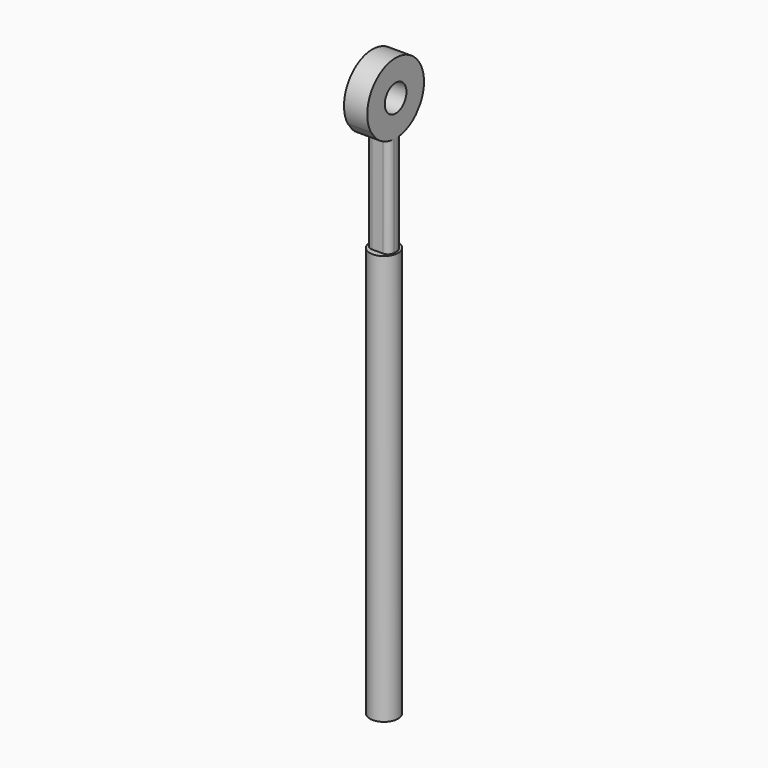
from build123d import *

# Parameters (mm, degrees)
F0_R         = 1.778
F1_DEPTH     = 51.562
F2_W         = 2.9239974657
F2_H         = 2.0237032442
F3_DEPTH     = 12.7
F4_R         = 1.7034886821
F5_DEPTH     = 2.92354
F6_T4_DEPTH  = 14.605
F6_S5_R      = 4.4583340214
F6_T6_DEPTH  = 9
F6_T10_DEPTH = 14.605
F6_S11_R     = 4.4583340214
F6_T12_DEPTH = 9
F6_T16_DEPTH = 14.605
F6_S17_R     = 4.4583340214
F6_T18_DEPTH = 9
F6_T22_DEPTH = 14.605
F6_S23_R     = 4.4583340214
F6_T24_DEPTH = 9


# Not quite as in the source:
# - a fillet or chamfer that OpenCascade refuses, or shapes differently, is made with other operations: its cross-section is extruded or revolved along the edge and cut away or added


with BuildPart() as f1:
    # F0 (on Top) → F1 (new body)
    with BuildSketch(Plane.XY):
        Circle(F0_R)
    extrude(amount=F1_DEPTH)

    # F2 (on face) → F3 (join)
    with BuildSketch(Plane.XY.offset(51.562)):
        Rectangle(F2_W, F2_H)
    extrude(amount=F3_DEPTH)

    # F4 (on face) → F5 (join)
    with BuildSketch(Plane.YZ.offset(1.4619987328)):
        with BuildLine():
            ThreePointArc((3.8834322811, 66.4140847097), (4.3122140778, 67.4719359292), (4.4583340214, 68.6039924622))
            ThreePointArc((4.4583340214, 68.6039924622), (-1.132056533, 72.91620654), (-3.8834322811, 66.4140847097))
            add(Edge.make_bspline(
                [(-3.1221140478, 65.4213605138), (-3.3692442223, 65.7498568477), (-3.6264069605, 66.0819292585), (-3.8834322811, 66.4140847097)],
                knots=[0.8083200784, 0.8083200784, 0.8083200784, 0.8083200784, 1, 1, 1, 1], degree=3))
            ThreePointArc((-3.1221140478, 65.4213605138), (-2.1467294288, 64.6965258908), (-1.0118516221, 64.262))
            Line((-1.0118516221, 64.262), (1.0118516221, 64.262))
            ThreePointArc((1.0118516221, 64.262), (2.1467294288, 64.6965258908), (3.1221140478, 65.4213605138))
            add(Edge.make_bspline(
                [(3.1221140478, 65.4213605138), (3.3692442223, 65.7498568477), (3.6264069605, 66.0819292585), (3.8834322811, 66.4140847097)],
                knots=[0.8083200784, 0.8083200784, 0.8083200784, 0.8083200784, 1, 1, 1, 1], degree=3))
        make_face()
        with Locations((0, 68.6039924622)):
            Circle(F4_R, mode=Mode.SUBTRACT)
    extrude(amount=-F5_DEPTH)

    # F6: fillet of radius 0.762 on 4 edges, made by hand


with BuildPart() as f6_tool2:
    # F6_s3 → F6_t4 (new body)
    with BuildSketch(Plane.XY.offset(51.562)):
        with BuildLine():
            ThreePointArc((1.4619987328, -0.2498516221), (1.2388141001, -0.7886669894), (0.6999987328, -1.0118516221))
            Line((0.6999987328, -1.0118516221), (1.4619987328, -1.0118516221))
            Line((1.4619987328, -1.0118516221), (1.4619987328, -0.2498516221))
        make_face()
    extrude(amount=F6_T4_DEPTH)

    # F6_s5 → F6_t6 (cut, symmetric)
    with BuildSketch(Plane.YZ.offset(1.1)):
        with Locations((0, 68.6039924622)):
            Circle(F6_S5_R)
    extrude(amount=F6_T6_DEPTH, both=True, mode=Mode.SUBTRACT)


with BuildPart() as f1_1:
    add(f1.part)

    # F6_t1: cut F6_tool2
    add(f6_tool2.part, mode=Mode.SUBTRACT)


with BuildPart() as f6_tool8:
    # F6_s9 → F6_t10 (new body)
    with BuildSketch(Plane.XY.offset(51.562)):
        with BuildLine():
            ThreePointArc((-1.4619987328, 0.2498516221), (-1.2388141001, 0.7886669894), (-0.6999987328, 1.0118516221))
            Line((-0.6999987328, 1.0118516221), (-1.4619987328, 1.0118516221))
            Line((-1.4619987328, 1.0118516221), (-1.4619987328, 0.2498516221))
        make_face()
    extrude(amount=F6_T10_DEPTH)

    # F6_s11 → F6_t12 (cut, symmetric)
    with BuildSketch(Plane.YZ.offset(-1.1)):
        with Locations((0, 68.6039924622)):
            Circle(F6_S11_R)
    extrude(amount=F6_T12_DEPTH, both=True, mode=Mode.SUBTRACT)


with BuildPart() as f1_2:
    add(f1_1.part)

    # F6_t7: cut F6_tool8
    add(f6_tool8.part, mode=Mode.SUBTRACT)


with BuildPart() as f6_tool14:
    # F6_s15 → F6_t16 (new body)
    with BuildSketch(Plane.XY.offset(51.562)):
        with BuildLine():
            ThreePointArc((1.4619987328, 0.2498516221), (1.2388141001, 0.7886669894), (0.6999987328, 1.0118516221))
            Line((0.6999987328, 1.0118516221), (1.4619987328, 1.0118516221))
            Line((1.4619987328, 1.0118516221), (1.4619987328, 0.2498516221))
        make_face()
    extrude(amount=F6_T16_DEPTH)

    # F6_s17 → F6_t18 (cut, symmetric)
    with BuildSketch(Plane.YZ.offset(1.1)):
        with Locations((0, 68.6039924622)):
            Circle(F6_S17_R)
    extrude(amount=F6_T18_DEPTH, both=True, mode=Mode.SUBTRACT)


with BuildPart() as f1_3:
    add(f1_2.part)

    # F6_t13: cut F6_tool14
    add(f6_tool14.part, mode=Mode.SUBTRACT)


with BuildPart() as f6_tool20:
    # F6_s21 → F6_t22 (new body)
    with BuildSketch(Plane.XY.offset(51.562)):
        with BuildLine():
            ThreePointArc((-0.6999987328, -1.0118516221), (-1.2388141001, -0.7886669894), (-1.4619987328, -0.2498516221))
            Line((-1.4619987328, -0.2498516221), (-1.4619987328, -1.0118516221))
            Line((-1.4619987328, -1.0118516221), (-0.6999987328, -1.0118516221))
        make_face()
    extrude(amount=F6_T22_DEPTH)

    # F6_s23 → F6_t24 (cut, symmetric)
    with BuildSketch(Plane.YZ.offset(-1.1)):
        with Locations((0, 68.6039924622)):
            Circle(F6_S23_R)
    extrude(amount=F6_T24_DEPTH, both=True, mode=Mode.SUBTRACT)


with BuildPart() as f1_4:
    add(f1_3.part)

    # F6_t19: cut F6_tool20
    add(f6_tool20.part, mode=Mode.SUBTRACT)


solid = f1_4.part
